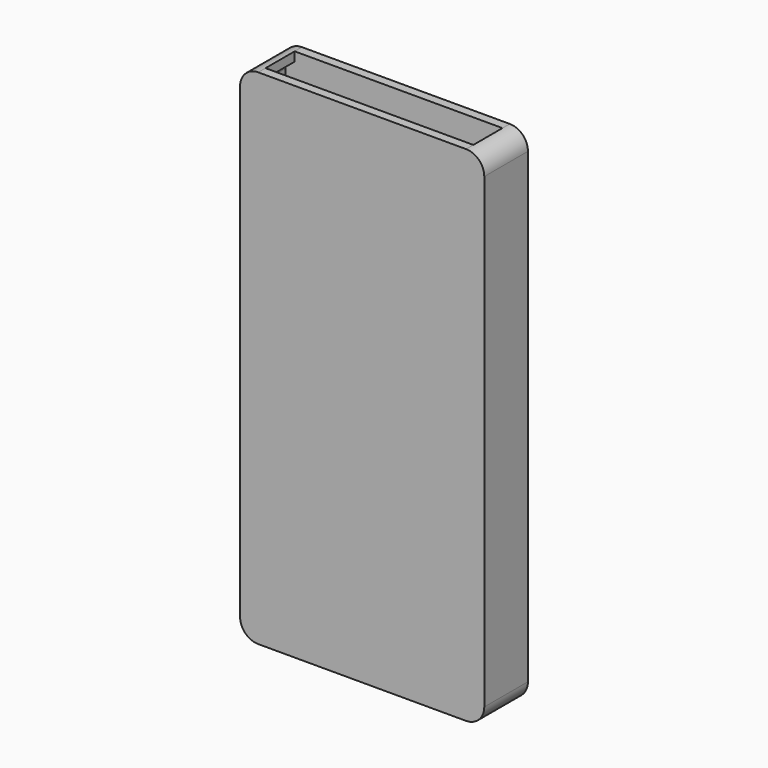
from build123d import *

# Parameters (mm, degrees)
F0_W     = 67.1
F0_H     = 138.3
F1_DEPTH = 15
F2_R     = 5
F3_T     = -2.5


# Not quite as in the source:
# - a shell that OpenCascade refuses in one call is made with other operations: the cavity is built on its own and cut out


with BuildPart() as f1:
    # F0 (on Front) → F1 (new body)
    with BuildSketch(Plane.XZ):
        Rectangle(F0_W, F0_H)
    extrude(amount=-F1_DEPTH)

    # F2
    f2_edges = [f1.edges().sort_by_distance(p)[0] for p in [
        (-33.55, 7.5, 69.15),
        (33.55, 7.5, 69.15),
        (-33.55, 7.5, -69.15),
        (33.55, 7.5, -69.15),
    ]]
    fillet(f2_edges, radius=F2_R)

    # F3: a shell. OpenCascade refuses it in one call, so the cavity is built on its own and cut out:
    # the body offset inwards by the wall thickness, plus a prism from it out through each open face.
    f3_core = offset(f1.part, amount=F3_T, mode=Mode.PRIVATE)
    f3_exits = [f3_core.faces().sort_by_distance(p)[0] for p in [
        (0, 7.5, 66.65),
    ]]
    add(f3_core, mode=Mode.SUBTRACT)
    extrude(f3_exits, amount=-F3_T, mode=Mode.SUBTRACT)


solid = f1.part
